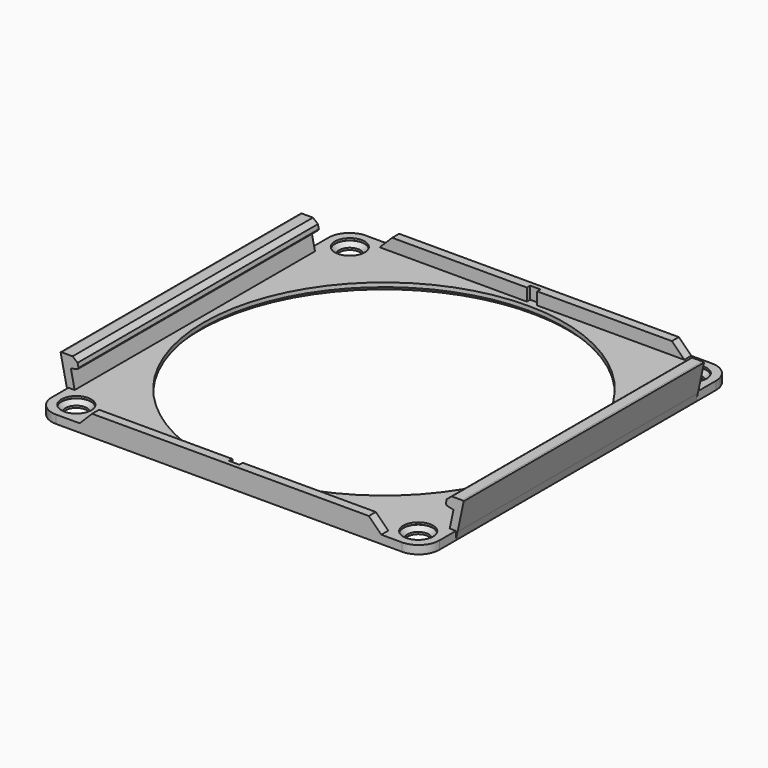
from build123d import *

# Parameters (mm, degrees)
F0_W       = 93.5
F0_H       = 93.5
F0_R       = 2.55
F0_R_2     = 43.5
F1_DEPTH   = 2
F3_START   = -10
F3_DEPTH   = 72.5
F4_SIZE    = 1
F6_DEPTH   = 3
F7_SIZE    = 2.99999
F8_R       = 3.6
F9_DEPTH   = 0.5
F10_SIZE   = 1
F11_R      = 5
F12_SIZE   = 1
F13_SIZE   = 0.3
F14_DEPTH  = 0.4
F15_DEPTH  = 0.4
F15_FACE_W = 0.4
F15_FACE_H = 72.5
F14_FACE_W = 0.4
F14_FACE_H = 72.5


# Not quite as in the source:
# - a fillet or chamfer is up to 0.001 mm smaller than in the source, because OpenCascade refuses the exact size


with BuildPart() as f1:
    # F0 (on Top) → F1 (new body)
    with BuildSketch(Plane.XY):
        with Locations((29.9444539048, 32.1819351325)):
            Rectangle(F0_W, F0_H)
        with Locations((-11.3055460952, -9.0680648675)):
            Circle(F0_R, mode=Mode.SUBTRACT)
        with Locations((71.1944539048, -9.0680648675)):
            Circle(F0_R, mode=Mode.SUBTRACT)
        with Locations((29.9444539048, 32.1819351325)):
            Circle(F0_R_2, mode=Mode.SUBTRACT)
        with Locations((-11.3055460952, 73.4319351325)):
            Circle(F0_R, mode=Mode.SUBTRACT)
        with Locations((71.1944539048, 73.4319351325)):
            Circle(F0_R, mode=Mode.SUBTRACT)
    extrude(amount=F1_DEPTH)

    # F2 (on face) → F3 (join)
    with BuildSketch(Plane.XZ.offset(14.5680648675).offset(F3_START)):
        Polygon((-16.8055460952, 9), (-16.2269746666, 6.3), (-14.3147795447, 6.7097560976), (-14.8055460952, 9), align=None)
        Polygon((-16.8055460952, 2), (-15.3055460952, 2), (-16.2269746666, 6.3), (-16.8055460952, 9), (-18.3055460952, 9), align=None)
        Polygon((76.1158824762, 6.3), (75.1944539048, 2), (76.6944539048, 2), (78.1944539048, 9), (76.6944539048, 9), align=None)
        Polygon((74.2036873543, 6.7097560976), (76.1158824762, 6.3), (76.6944539048, 9), (74.6944539048, 9), align=None)
    extrude(amount=-F3_DEPTH)

    # F4
    f4_edges = [f1.edges().sort_by_distance(p)[0] for p in [
        (-14.805546, 31.681935, 9),
        (74.694454, 31.681935, 9),
    ]]
    chamfer(f4_edges, length=F4_SIZE)

    # F5 (on face) → F6 (join)
    with BuildSketch(Plane.XY.offset(2)):
        Polygon((-6.0960170065, -14.5680648675), (66.6944539048, -14.5680648675), (66.6944539048, -12.4680648675), (31.5492184492, -12.4680648675), (31.5492184492, -13.4680648675), (29.0492184492, -13.4680648675), (29.0492184492, -12.4680648675), (-6.0960170065, -12.4680648675), align=None)
        Polygon((66.6944539048, 76.8319351325), (66.6944539048, 78.9319351325), (-6.8055460952, 78.9319351325), (-6.8055460952, 76.8319351325), (28.6944539048, 76.8319351325), (28.6944539048, 77.8319351325), (31.1944539048, 77.8319351325), (31.1944539048, 76.8319351325), align=None)
    extrude(amount=F6_DEPTH)

    # F7 (size 3 in the source; OpenCascade refuses exactly that, so slightly less here)
    f7_edges = [f1.edges().sort_by_distance(p)[0] for p in [
        (66.694454, -13.518065, 5),
        (-6.096017, -13.518065, 5),
        (-6.805546, 77.881935, 5),
        (66.694454, 77.881935, 5),
    ]]
    chamfer(f7_edges, length=F7_SIZE)

    # F8 (on face) → F9 (cut)
    with BuildSketch(Plane.XY.offset(2)):
        with Locations((-11.3055460952, -9.0680648675)):
            Circle(F8_R)
        with Locations((71.1944539048, -9.0680648675)):
            Circle(F8_R)
        with Locations((71.1944539048, 73.4319351325)):
            Circle(F8_R)
        with Locations((-11.3055460952, 73.4319351325)):
            Circle(F8_R)
    extrude(amount=-F9_DEPTH, mode=Mode.SUBTRACT)

    # F10
    f10_edges = [f1.edges().sort_by_distance(p)[0] for p in [
        (-13.855546, -9.068065, 1.5),
        (68.644454, -9.068065, 1.5),
        (68.644454, 73.431935, 1.5),
        (-13.855546, 73.431935, 1.5),
    ]]
    chamfer(f10_edges, length=F10_SIZE)

    # F11
    f11_edges = [f1.edges().sort_by_distance(p)[0] for p in [
        (-16.805546, 78.931935, 1),
        (-16.805546, -14.568065, 1),
        (76.694454, -14.568065, 1),
        (76.694454, 78.931935, 1),
    ]]
    fillet(f11_edges, radius=F11_R)

    # F12
    f12_edges = [f1.edges().sort_by_distance(p)[0] for p in [
        (-13.555546, 32.181935, 0),
    ]]
    chamfer(f12_edges, length=F12_SIZE)

    # F13
    f13_edges = [f1.edges().sort_by_distance(p)[0] for p in [
        (-14.31478, 31.681935, 6.709756),
        (74.203687, 31.681935, 6.709756),
    ]]
    chamfer(f13_edges, length=F13_SIZE)

    # F14 (add): a face of the model
    f14_faces = [f1.faces().sort_by_distance(p)[0] for p in [
        (-17.5555460952, 31.6819351325, 5.5),
    ]]
    extrude(f14_faces, amount=F14_DEPTH)

    # F15 (add): a face of the model
    f15_faces = [f1.faces().sort_by_distance(p)[0] for p in [
        (77.4444539048, 31.6819351325, 5.5),
    ]]
    extrude(f15_faces, amount=F15_DEPTH)

    # F15_face (on face) → F16 (join, up to the next surface of F1)
    with BuildSketch(Plane(origin=(76.8900143876, 31.6819351325, 1.9580941823), x_dir=(1, 0, 0), z_dir=(-0.2095290887, 0, -0.9778024141))):
        Rectangle(F15_FACE_W, F15_FACE_H)
    extrude(until=Until.NEXT)

    # F14_face (on face) → F17 (join, up to the next surface of F1)
    with BuildSketch(Plane(origin=(-17.001106578, 31.6819351325, 1.9580941823), x_dir=(1, 0, 0), z_dir=(0.2095290887, 0, -0.9778024141))):
        Rectangle(F14_FACE_W, F14_FACE_H)
    extrude(until=Until.NEXT)


solid = f1.part
